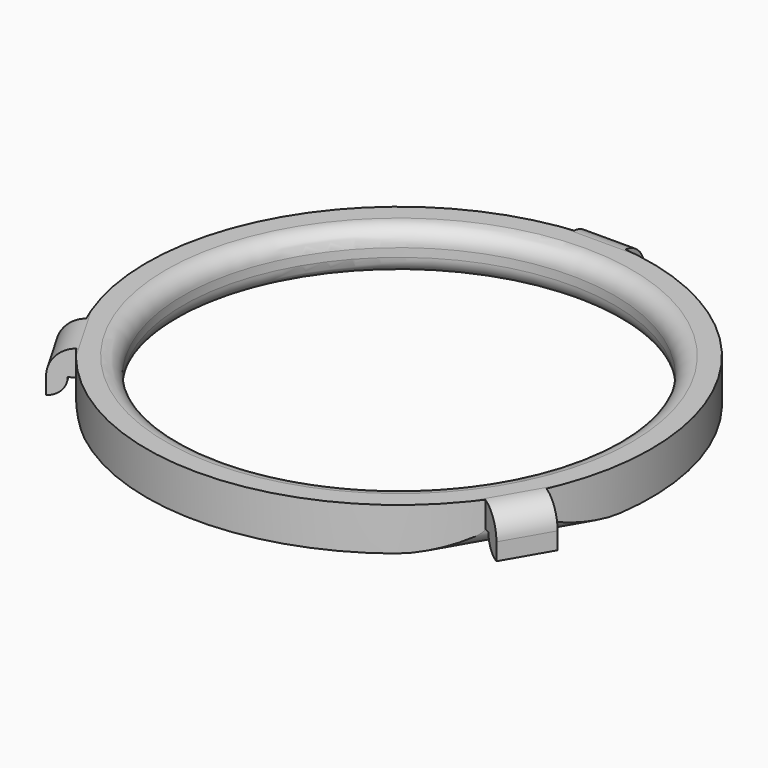
from build123d import *

# Parameters (mm, degrees)
F0_R     = 29.5
F0_R_2   = 25.25
F1_DEPTH = 5
F3_W     = 6
F3_H     = 5
F4_DEPTH = 5
F5_R     = 3
F6_W     = 6
F6_H     = 0.7910079116
F7_DEPTH = 2
F8_R     = 1.99999


# Not quite as in the source:
# - a fillet or chamfer is up to 0.001 mm smaller than in the source, because OpenCascade refuses the exact size
# - a feature of the source that left no trace in its solid (it failed there, or was rolled back) is left out


with BuildPart() as f1:
    # F0 (on Top) → F1 (new body)
    with BuildSketch(Plane.XY):
        Circle(F0_R)
        Circle(F0_R_2, mode=Mode.SUBTRACT)
    extrude(amount=F1_DEPTH)

    # F3 (on Top) → F4 (join)
    with BuildSketch(Plane.XY):
        with Locations((0, 29.6380690932)):
            Rectangle(F3_W, F3_H)
        Polygon((-29.3323842633, -13.4709583353), (-26.3323842633, -18.667110758), (-22.0022572444, -16.167110758), (-25.0022572444, -10.9709583353), align=None)
        Polygon((26.3323842633, -18.667110758), (29.3323842633, -13.4709583353), (25.0022572444, -10.9709583353), (22.0022572444, -16.167110758), align=None)
    extrude(amount=F4_DEPTH)

    # F5
    f5_edges = [f1.edges().sort_by_distance(p)[0] for p in [
        (0, 32.138069, 5),
        (-27.832384, -16.069035, 5),
        (27.832384, -16.069035, 5),
    ]]
    fillet(f5_edges, radius=F5_R)

    # F6 (on face) → F7 (cut)
    with BuildSketch(Plane(origin=(0, 0, 0), x_dir=(1, 0, 0), z_dir=(0, 0, -1))):
        with Locations((0, -29.7425651374)):
            Rectangle(F6_W, F6_H)
        Polygon((24.6003334557, 17.667110758), (23.9153005097, 17.2716068022), (26.9153005097, 12.0754543795), (27.6003334557, 12.4709583353), align=None)
        Polygon((-27.6003334557, 12.4709583353), (-26.9153005097, 12.0754543795), (-23.9153005097, 17.2716068022), (-24.6003334557, 17.667110758), align=None)
    extrude(amount=-F7_DEPTH, mode=Mode.SUBTRACT)

    # F8 (radius 2 in the source; OpenCascade refuses exactly that, so slightly less here)
    f8_edges = [f1.edges().sort_by_distance(p)[0] for p in [
        (0, 29.347061, 0),
        (0, 30.138069, 0),
        (26.100333, -15.069035, 0),
        (25.415301, -14.673531, 0),
        (-25.415301, -14.673531, 0),
        (-26.100333, -15.069035, 0),
        (-25.25, 0, 0),
        (-25.25, 0, 5),
    ]]
    fillet(f8_edges, radius=F8_R)


solid = f1.part
